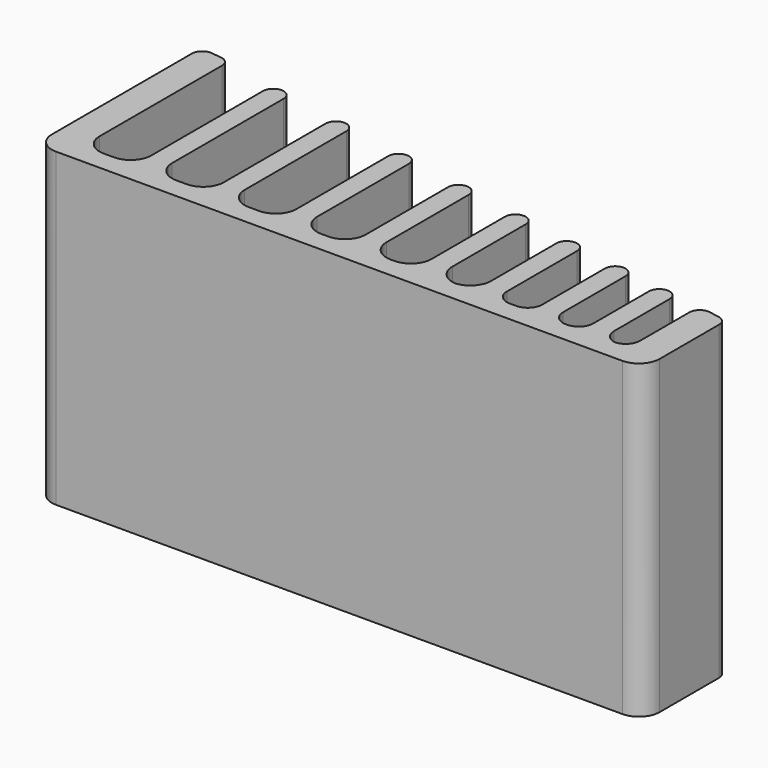
from build123d import *

# Parameters (mm, degrees)
F1_DEPTH    = 38.1
F2_T1_DEPTH = 38.1
F2_T3_DEPTH = 50.8
F3_T1_DEPTH = 38.1
F4_R        = 1.26999


# Not quite as in the source:
# - a fillet or chamfer that OpenCascade refuses, or shapes differently, is made with other operations: its cross-section is extruded or revolved along the edge and cut away or added
# - a fillet or chamfer is up to 0.001 mm smaller than in the source, because OpenCascade refuses the exact size


with BuildPart() as f1:
    # F0 (on Top) → F1 (new body)
    with BuildSketch(Plane.XY):
        Polygon((-37.2364, 25.4), (-37.2364, 0), (37.2364, 0), (37.2364, 12.7), (33.4264, 13.3497271487), (33.4264, 2.54), (30.226, 2.54), (30.226, 13.8954979536), (27.686, 14.3286493861), (27.686, 2.54), (23.9776, 2.54), (23.9776, 14.9610504775), (21.4376, 15.39420191), (21.4376, 2.54), (17.0942, 2.54), (17.0942, 16.1348908595), (14.5542, 16.568042292), (14.5542, 2.54), (9.8044, 2.54), (9.8044, 17.3780354707), (7.2644, 17.8111869031), (7.2644, 2.54), (1.7272, 2.54), (1.7272, 18.7554570259), (-0.8128, 19.1886084584), (-0.8128, 2.54), (-6.7564, 2.54), (-6.7564, 20.2021828104), (-9.2964, 20.6353342428), (-9.2964, 2.54), (-15.6464, 2.54), (-15.6464, 21.718212824), (-18.1864, 22.1513642565), (-18.1864, 2.54), (-24.5364, 2.54), (-24.5364, 23.2342428377), (-27.0764, 23.6673942701), (-27.0764, 2.54), (-33.4264, 2.54), (-33.4264, 24.9766666667), align=None)
    extrude(amount=F1_DEPTH)

    # F2: fillet of radius 2.54 on 14 edges, made by hand

    # F2_s2 → F2_t1 (join)
    with BuildSketch(Plane.XY):
        with BuildLine():
            ThreePointArc((-30.8864, 2.54), (-32.6824512242, 3.2839487758), (-33.4264, 5.08))
            Line((-33.4264, 5.08), (-33.4264, 2.54))
            Line((-33.4264, 2.54), (-30.8864, 2.54))
        make_face()
        with BuildLine():
            ThreePointArc((-27.0764, 5.08), (-27.8203487758, 3.2839487758), (-29.6164, 2.54))
            Line((-29.6164, 2.54), (-27.0764, 2.54))
            Line((-27.0764, 2.54), (-27.0764, 5.08))
        make_face()
        with BuildLine():
            ThreePointArc((-21.9964, 2.54), (-23.7924512242, 3.2839487758), (-24.5364, 5.08))
            Line((-24.5364, 5.08), (-24.5364, 2.54))
            Line((-24.5364, 2.54), (-21.9964, 2.54))
        make_face()
        with BuildLine():
            ThreePointArc((-18.1864, 5.08), (-18.9303487758, 3.2839487758), (-20.7264, 2.54))
            Line((-20.7264, 2.54), (-18.1864, 2.54))
            Line((-18.1864, 2.54), (-18.1864, 5.08))
        make_face()
        with BuildLine():
            ThreePointArc((-13.1064, 2.54), (-14.9024512242, 3.2839487758), (-15.6464, 5.08))
            Line((-15.6464, 5.08), (-15.6464, 2.54))
            Line((-15.6464, 2.54), (-13.1064, 2.54))
        make_face()
        with BuildLine():
            ThreePointArc((-9.2964, 5.08), (-10.0403487758, 3.2839487758), (-11.8364, 2.54))
            Line((-11.8364, 2.54), (-9.2964, 2.54))
            Line((-9.2964, 2.54), (-9.2964, 5.08))
        make_face()
        with BuildLine():
            ThreePointArc((-4.2164, 2.54), (-6.0124512242, 3.2839487758), (-6.7564, 5.08))
            Line((-6.7564, 5.08), (-6.7564, 2.54))
            Line((-6.7564, 2.54), (-4.2164, 2.54))
        make_face()
        with BuildLine():
            ThreePointArc((-0.8128, 5.08), (-1.5567487758, 3.2839487758), (-3.3528, 2.54))
            Line((-3.3528, 2.54), (-0.8128, 2.54))
            Line((-0.8128, 2.54), (-0.8128, 5.08))
        make_face()
        with BuildLine():
            ThreePointArc((4.2672, 2.54), (2.4711487758, 3.2839487758), (1.7272, 5.08))
            Line((1.7272, 5.08), (1.7272, 2.54))
            Line((1.7272, 2.54), (4.2672, 2.54))
        make_face()
        with BuildLine():
            ThreePointArc((7.2644, 5.08), (6.5204512242, 3.2839487758), (4.7244, 2.54))
            Line((4.7244, 2.54), (7.2644, 2.54))
            Line((7.2644, 2.54), (7.2644, 5.08))
        make_face()
        with BuildLine():
            ThreePointArc((12.3444, 2.54), (10.5483487758, 3.2839487758), (9.8044, 5.08))
            Line((9.8044, 5.08), (9.8044, 2.54))
            Line((9.8044, 2.54), (12.3444, 2.54))
        make_face()
        with BuildLine():
            ThreePointArc((14.5542, 5.08), (13.8102512242, 3.2839487758), (12.0142, 2.54))
            Line((12.0142, 2.54), (14.5542, 2.54))
            Line((14.5542, 2.54), (14.5542, 5.08))
        make_face()
    extrude(amount=F2_T1_DEPTH)

    # F2_s4 → F2_t3 (cut)
    with BuildSketch(Plane.XY.offset(-6.35)):
        with BuildLine():
            ThreePointArc((-37.2364, 2.54), (-36.4924512242, 0.7439487758), (-34.6964, 0))
            Line((-34.6964, 0), (-37.2364, 0))
            Line((-37.2364, 0), (-37.2364, 2.54))
        make_face()
        with BuildLine():
            ThreePointArc((34.6964, 0), (36.4924512242, 0.7439487758), (37.2364, 2.54))
            Line((37.2364, 2.54), (37.2364, 0))
            Line((37.2364, 0), (34.6964, 0))
        make_face()
    extrude(amount=F2_T3_DEPTH, mode=Mode.SUBTRACT)

    # F3: fillet of radius 1.778 on 6 edges, made by hand

    # F3_s2 → F3_t1 (join)
    with BuildSketch(Plane.XY):
        with BuildLine():
            ThreePointArc((17.0942, 4.318), (17.6149641431, 3.0607641431), (18.8722, 2.54))
            Line((18.8722, 2.54), (17.0942, 2.54))
            Line((17.0942, 2.54), (17.0942, 4.318))
        make_face()
        with BuildLine():
            ThreePointArc((19.6596, 2.54), (20.9168358569, 3.0607641431), (21.4376, 4.318))
            Line((21.4376, 4.318), (21.4376, 2.54))
            Line((21.4376, 2.54), (19.6596, 2.54))
        make_face()
        with BuildLine():
            ThreePointArc((23.9776, 4.318), (24.4983641431, 3.0607641431), (25.7556, 2.54))
            Line((25.7556, 2.54), (23.9776, 2.54))
            Line((23.9776, 2.54), (23.9776, 4.318))
        make_face()
        with BuildLine():
            ThreePointArc((25.908, 2.54), (27.1652358569, 3.0607641431), (27.686, 4.318))
            Line((27.686, 4.318), (27.686, 2.54))
            Line((27.686, 2.54), (25.908, 2.54))
        make_face()
        with BuildLine():
            ThreePointArc((30.226, 4.318), (30.7467641431, 3.0607641431), (32.004, 2.54))
            Line((32.004, 2.54), (30.226, 2.54))
            Line((30.226, 2.54), (30.226, 4.318))
        make_face()
        with BuildLine():
            ThreePointArc((31.6484, 2.54), (32.9056358569, 3.0607641431), (33.4264, 4.318))
            Line((33.4264, 4.318), (33.4264, 2.54))
            Line((33.4264, 2.54), (31.6484, 2.54))
        make_face()
    extrude(amount=F3_T1_DEPTH)

    # F4 (radius 1.27 in the source; OpenCascade refuses exactly that, so slightly less here)
    f4_edges = [f1.edges().sort_by_distance(p)[0] for p in [
        (33.4264, 13.349727, 19.05),
        (30.226, 13.895498, 19.05),
        (27.686, 14.328649, 19.05),
        (23.9776, 14.96105, 19.05),
        (21.4376, 15.394202, 19.05),
        (17.0942, 16.134891, 19.05),
        (14.5542, 16.568042, 19.05),
        (9.8044, 17.378035, 19.05),
        (7.2644, 17.811187, 19.05),
        (1.7272, 18.755457, 19.05),
        (-0.8128, 19.188608, 19.05),
        (-6.7564, 20.202183, 19.05),
        (-15.6464, 21.718213, 19.05),
        (-24.5364, 23.234243, 19.05),
        (-27.0764, 23.667394, 19.05),
        (-33.4264, 24.976667, 19.05),
        (-37.2364, 25.4, 19.05),
        (37.2364, 12.7, 19.05),
        (-9.2964, 20.635334, 19.05),
        (-18.1864, 22.151364, 19.05),
    ]]
    fillet(f4_edges, radius=F4_R)


solid = f1.part
